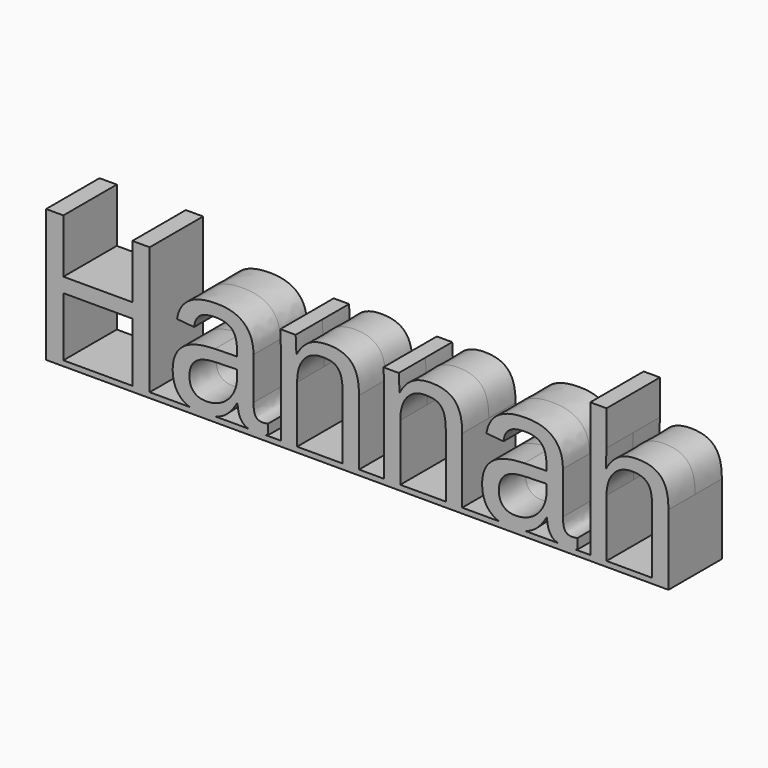
from build123d import *

# Parameters (mm, degrees)
F0_TEXT_SIZE = 35.2777777778
F1_DEPTH     = 6.35
F2_W         = 118.3845052083
F2_H         = 12.7
F3_DEPTH     = 1


# Not quite as in the source:
# - Text() gives the source's letters only with a copy of the font that has no kerning and outlines rounded to 1/6400 em; it was checked with that copy


with BuildPart() as f1:
    # F0 (on Front) → F1 (new body, symmetric)
    with BuildSketch(Plane.XZ):
        with Locations((-61.862890625, 0)):
            Text('Hannah', F0_TEXT_SIZE, font='Arimo', text_align=(TextAlign.LEFT, TextAlign.BOTTOM))
    extrude(amount=F1_DEPTH, both=True)

    # F2 (on Top) → F3 (join)
    with BuildSketch(Plane.XY):
        with Locations((0.2232421875, 0)):
            Rectangle(F2_W, F2_H)
    extrude(amount=-F3_DEPTH)


solid = f1.part
